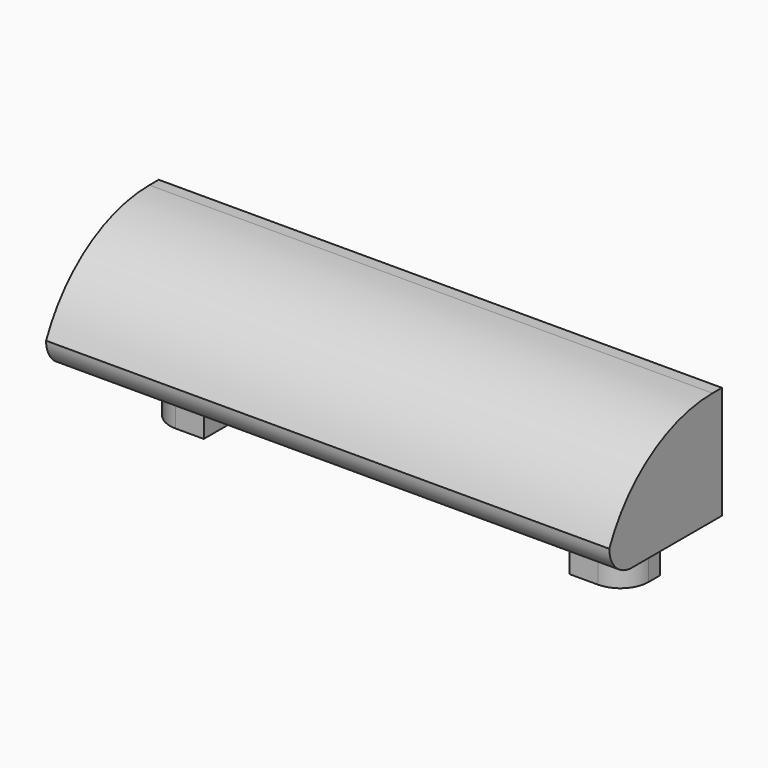
from build123d import *

# Parameters (mm, degrees)
F0_W        = 50.8
F0_H        = 12.7
F1_DEPTH    = 10.16
F2_W        = 5.08
F2_H        = 3.81
F3_DEPTH    = 5.08
F4_W        = 5.08
F4_H        = 3.81
F5_DEPTH    = 5.08
F6_R        = 2.54
F7_T1_DEPTH = 108.9987113259


# Not quite as in the source:
# - a fillet or chamfer that OpenCascade refuses, or shapes differently, is made with other operations: its cross-section is extruded or revolved along the edge and cut away or added


with BuildPart() as f1:
    # F0 (on Top) → F1 (new body)
    with BuildSketch(Plane.XY):
        with Locations((25.4, 6.35)):
            Rectangle(F0_W, F0_H)
    extrude(amount=F1_DEPTH)

    # F2 (on face) → F3 (join)
    with BuildSketch(Plane(origin=(0, 0, 0), x_dir=(1, 0, 0), z_dir=(0, 0, -1))):
        with Locations((6.35, -8.5725)):
            Rectangle(F2_W, F2_H)
    extrude(amount=F3_DEPTH)

    # F4 (on face) → F5 (join)
    with BuildSketch(Plane(origin=(0, 0, 0), x_dir=(1, 0, 0), z_dir=(0, 0, -1))):
        with Locations((44.45, -8.5598)):
            Rectangle(F4_W, F4_H)
    extrude(amount=F5_DEPTH)

    # F6
    f6_edges = [f1.edges().sort_by_distance(p)[0] for p in [
        (3.81, 6.6675, -2.54),
        (46.99, 6.6548, -2.54),
        (25.4, 0, 0),
    ]]
    fillet(f6_edges, radius=F6_R)

    # F7: fillet of radius 12.7 on 1 edges, made by hand

    # F7_s2 → F7_t1 (cut)
    with BuildSketch(Plane.YZ.offset(-29.099355663)):
        with BuildLine():
            ThreePointArc((0, 2.54), (4.6836657849, 8.085582337), (11.6397422652, 10.16))
            Line((11.6397422652, 10.16), (0, 10.16))
            Line((0, 10.16), (0, 2.54))
        make_face()
    extrude(amount=F7_T1_DEPTH, mode=Mode.SUBTRACT)


solid = f1.part
